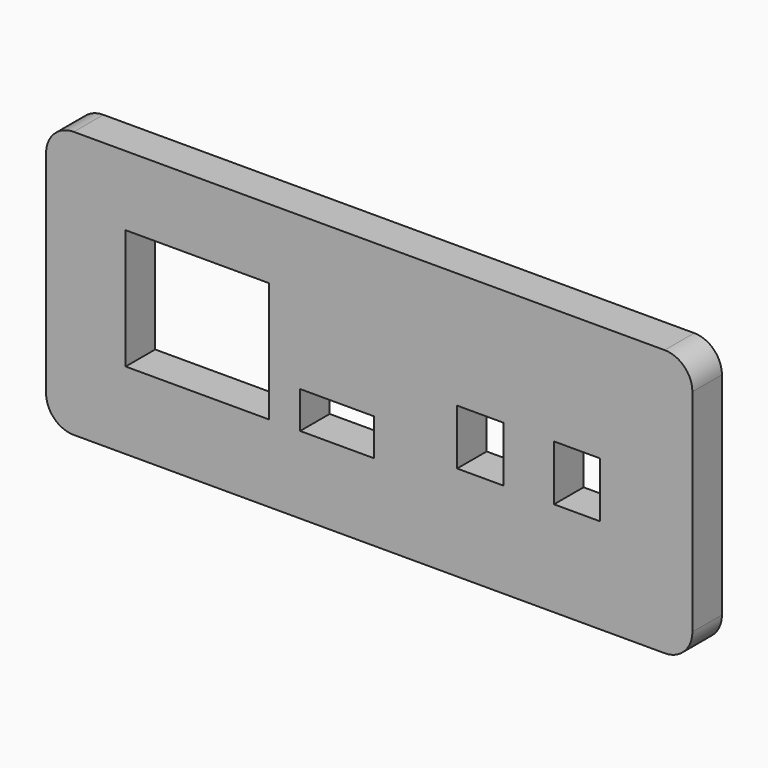
from build123d import *

# Parameters (mm, degrees)
F0_W     = 8
F0_H     = 4
F0_W_2   = 5
F0_H_2   = 6
F0_W_3   = 15.5
F0_H_3   = 13
F1_DEPTH = 1.8
F2_DEPTH = 2
F3_DEPTH = 2


# Not quite as in the source:
# - a feature of the source that left no trace in its solid (it failed there, or was rolled back) is left out


with BuildPart() as f1:
    # F0 (on Front) → F1 (new body)
    with BuildSketch(Plane.XZ):
        with BuildLine():
            Line((34.7865003794, 6.2641621617), (-29.2134996206, 6.2641621617))
            ThreePointArc((-29.2134996206, 6.2641621617), (-31.3348199641, 5.3854825052), (-32.2134996206, 3.2641621617))
            Line((-32.2134996206, 3.2641621617), (-32.2134996206, -19.6358378383))
            ThreePointArc((-32.2134996206, -19.6358378383), (-31.3348199641, -21.7571581819), (-29.2134996206, -22.6358378383))
            Line((-29.2134996206, -22.6358378383), (34.7865003794, -22.6358378383))
            ThreePointArc((34.7865003794, -22.6358378383), (36.907820723, -21.7571581819), (37.7865003794, -19.6358378383))
            Line((37.7865003794, -19.6358378383), (37.7865003794, 3.2641621617))
            ThreePointArc((37.7865003794, 3.2641621617), (36.907820723, 5.3854825052), (34.7865003794, 6.2641621617))
        make_face()
        with Locations((-0.6956385732, -12.2858378383)):
            Rectangle(F0_W, F0_H, mode=Mode.SUBTRACT)
        with Locations((14.8043614268, -9.3358378383)):
            Rectangle(F0_W_2, F0_H_2, mode=Mode.SUBTRACT)
        with Locations((25.3043614268, -9.3358378383)):
            Rectangle(F0_W_2, F0_H_2, mode=Mode.SUBTRACT)
        with Locations((-15.8456385732, -7.7858378383)):
            Rectangle(F0_W_3, F0_H_3, mode=Mode.SUBTRACT)
    extrude(amount=F1_DEPTH)

    # F0 (on Front) → F2 (join)
    with BuildSketch(Plane.XZ):
        with BuildLine():
            Line((34.7865003794, 6.2641621617), (-29.2134996206, 6.2641621617))
            ThreePointArc((-29.2134996206, 6.2641621617), (-31.3348199641, 5.3854825052), (-32.2134996206, 3.2641621617))
            Line((-32.2134996206, 3.2641621617), (-32.2134996206, -19.6358378383))
            ThreePointArc((-32.2134996206, -19.6358378383), (-31.3348199641, -21.7571581819), (-29.2134996206, -22.6358378383))
            Line((-29.2134996206, -22.6358378383), (34.7865003794, -22.6358378383))
            ThreePointArc((34.7865003794, -22.6358378383), (36.907820723, -21.7571581819), (37.7865003794, -19.6358378383))
            Line((37.7865003794, -19.6358378383), (37.7865003794, 3.2641621617))
            ThreePointArc((37.7865003794, 3.2641621617), (36.907820723, 5.3854825052), (34.7865003794, 6.2641621617))
        make_face()
        with Locations((-0.6956385732, -12.2858378383)):
            Rectangle(F0_W, F0_H, mode=Mode.SUBTRACT)
        with Locations((14.8043614268, -9.3358378383)):
            Rectangle(F0_W_2, F0_H_2, mode=Mode.SUBTRACT)
        with Locations((25.3043614268, -9.3358378383)):
            Rectangle(F0_W_2, F0_H_2, mode=Mode.SUBTRACT)
        with Locations((-15.8456385732, -7.7858378383)):
            Rectangle(F0_W_3, F0_H_3, mode=Mode.SUBTRACT)
    extrude(amount=F2_DEPTH)

    # F3 (add): a face of the model
    f3_faces = [f1.faces().sort_by_distance(p)[0] for p in [
        (4.4299984424, -2, -8.1163746121),
    ]]
    extrude(f3_faces, amount=F3_DEPTH)


solid = f1.part
